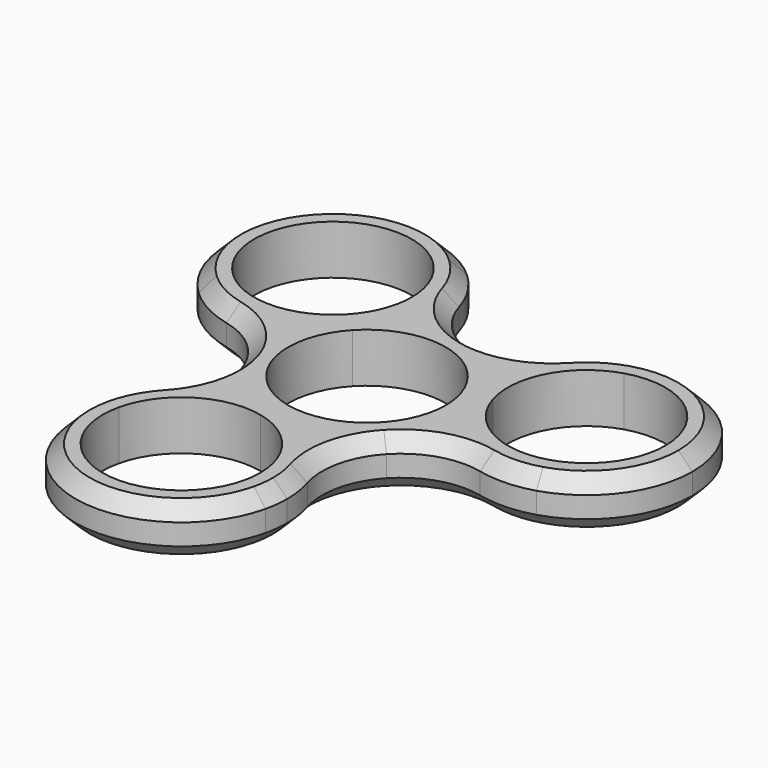
from build123d import *

# Parameters (mm, degrees)
F1_DEPTH = 7
F2_R     = 11.159
F3_SIZE  = 2


# Not quite as in the source:
# - a fillet or chamfer is up to 0.001 mm smaller than in the source, because OpenCascade refuses the exact size
# - ends of sketch curves that miss each other by under 0.0002 mm in the source are joined


with BuildPart() as f1:
    # F0 (on Top) → F1 (new body)
    with BuildSketch(Plane.XY):
        with BuildLine():
            Line((-29.35523, 6.900439), (-26.73352, 9.706189))
            ThreePointArc((-26.73352, 9.706189), (-27.268387, 25.479747), (-11.494829, 26.014613))
            Line((-11.494829, 26.014613), (-8.873119, 28.820364))
            ThreePointArc((-8.873119, 28.820364), (-30.074137, 28.101457), (-29.35523, 6.900439))
        make_face()
        with BuildLine():
            ThreePointArc((-8.873119, 28.820364), (-7.418015, 23.350137), (-4.139731, 18.735642))
            ThreePointArc((-4.139731, 18.735642), (-5.535487, 24.233724), (-8.873119, 28.820364))
        make_face()
        with BuildLine():
            ThreePointArc((-7.954175, 17.860401), (-8.732782, 13.765002), (-10.959962, 10.241056))
            ThreePointArc((-10.959962, 10.241056), (-8.01264, 12.680599), (-4.54403, 14.295167))
            ThreePointArc((-4.54403, 14.295167), (-4.222026, 16.064874), (-4.114175, 17.860401))
            ThreePointArc((-4.114175, 17.860401), (-4.120565, 18.298208), (-4.139731, 18.735642))
            ThreePointArc((-4.139731, 18.735642), (-7.418015, 23.350137), (-8.873119, 28.820364))
            Line((-8.873119, 28.820364), (-11.494829, 26.014613))
            ThreePointArc((-11.494829, 26.014613), (-8.877537, 22.305269), (-7.954175, 17.860401))
        make_face()
        with BuildLine():
            Line((-10.959962, 10.241056), (-8.154212, 7.619345))
            ThreePointArc((-8.154212, 7.619345), (-5.919925, 10.725153), (-4.54403, 14.295167))
            ThreePointArc((-4.54403, 14.295167), (-8.01264, 12.680599), (-10.959962, 10.241056))
        make_face()
        with BuildLine():
            ThreePointArc((-14.570144, 3.565235), (-11.101534, 5.179802), (-8.154212, 7.619345))
            Line((-8.154212, 7.619345), (-10.959962, 10.241056))
            ThreePointArc((-10.959962, 10.241056), (-13.19425, 7.135248), (-14.570144, 3.565235))
        make_face()
        with BuildLine():
            ThreePointArc((-14.570144, 3.565235), (-13.19425, 7.135248), (-10.959962, 10.241056))
            ThreePointArc((-10.959962, 10.241056), (-18.735967, 6.706812), (-26.73352, 9.706189))
            Line((-26.73352, 9.706189), (-29.35523, 6.900439))
            ThreePointArc((-29.35523, 6.900439), (-23.798999, 5.819232), (-18.973032, 2.861065))
            ThreePointArc((-18.973032, 2.861065), (-16.745277, 3.048638), (-14.570144, 3.565235))
        make_face()
        with BuildLine():
            ThreePointArc((-29.35523, 6.900439), (-24.553034, 3.881174), (-18.973032, 2.861065))
            ThreePointArc((-18.973032, 2.861065), (-23.798999, 5.819232), (-29.35523, 6.900439))
        make_face()
        with BuildLine():
            ThreePointArc((-20.522608, -22.094528), (-16.512804, -18.099258), (-14.155676, -12.952933))
            ThreePointArc((-14.155676, -12.952933), (-18.219277, -16.910735), (-20.522608, -22.094528))
        make_face()
        with BuildLine():
            ThreePointArc((-16.781901, -22.962121), (-11.814806, -16.013373), (-3.389033, -14.612134))
            ThreePointArc((-3.389033, -14.612134), (-6.975401, -13.27945), (-10.107962, -11.082829))
            ThreePointArc((-10.107962, -11.082829), (-12.201695, -11.86664), (-14.155676, -12.952933))
            ThreePointArc((-14.155676, -12.952933), (-16.512804, -18.099258), (-20.522608, -22.094528))
            Line((-20.522608, -22.094528), (-16.781901, -22.962121))
        make_face()
        with BuildLine():
            Line((-3.389033, -14.612134), (-2.521441, -10.871428))
            ThreePointArc((-2.521441, -10.871428), (-6.328293, -10.489382), (-10.107962, -11.082829))
            ThreePointArc((-10.107962, -11.082829), (-6.975401, -13.27945), (-3.389033, -14.612134))
        make_face()
        with BuildLine():
            ThreePointArc((4.197488, -14.400732), (1.064927, -12.204112), (-2.521441, -10.871428))
            Line((-2.521441, -10.871428), (-3.389033, -14.612134))
            ThreePointArc((-3.389033, -14.612134), (0.417819, -14.99418), (4.197488, -14.400732))
        make_face()
        with BuildLine():
            ThreePointArc((9.089526, -25.483561), (8.559988, -21.533151), (7.008761, -17.861661))
            ThreePointArc((7.008761, -17.861661), (6.859897, -23.520154), (8.70166, -28.872595))
            ThreePointArc((8.70166, -28.872595), (8.992244, -27.189139), (9.089526, -25.483561))
        make_face()
        with BuildLine():
            ThreePointArc((4.197488, -14.400732), (0.417819, -14.99418), (-3.389033, -14.612134))
            ThreePointArc((-3.389033, -14.612134), (2.826942, -18.540712), (5.249526, -25.483561))
            ThreePointArc((5.249526, -25.483561), (5.177148, -26.752511), (4.960954, -28.005002))
            Line((4.960954, -28.005002), (8.70166, -28.872595))
            ThreePointArc((8.70166, -28.872595), (6.859897, -23.520154), (7.008761, -17.861661))
            ThreePointArc((7.008761, -17.861661), (5.732441, -16.026155), (4.197488, -14.400732))
        make_face()
        with BuildLine():
            ThreePointArc((4.960954, -28.005002), (-8.431915, -36.354989), (-16.781901, -22.962121))
            Line((-16.781901, -22.962121), (-20.522608, -22.094528))
            ThreePointArc((-20.522608, -22.094528), (-9.299507, -40.095695), (8.70166, -28.872595))
            Line((8.70166, -28.872595), (4.960954, -28.005002))
        make_face()
        with BuildLine():
            ThreePointArc((-10.107962, -11.082829), (-6.328293, -10.489382), (-2.521441, -10.871428))
            ThreePointArc((-2.521441, -10.871428), (-10.675653, -3.252082), (-8.154212, 7.619345))
            ThreePointArc((-8.154212, 7.619345), (-11.101534, 5.179802), (-14.570144, 3.565235))
            ThreePointArc((-14.570144, 3.565235), (-14.99418, -0.417819), (-14.348996, -4.371078))
            ThreePointArc((-14.348996, -4.371078), (-12.680599, -8.01264), (-10.107962, -11.082829))
        make_face()
        with BuildLine():
            ThreePointArc((10.675653, 3.252082), (11.038249, 1.643976), (11.16, 0))
            ThreePointArc((11.16, 0), (6.94285, -8.737416), (-2.521441, -10.871428))
            ThreePointArc((-2.521441, -10.871428), (1.064927, -12.204112), (4.197488, -14.400732))
            ThreePointArc((4.197488, -14.400732), (7.858931, -12.776431), (10.959962, -10.241056))
            ThreePointArc((10.959962, -10.241056), (13.279449, -6.975401), (14.651993, -3.212338))
            ThreePointArc((14.651993, -3.212338), (12.248217, -0.235772), (10.675653, 3.252082))
        make_face()
        with BuildLine():
            Line((14.348996, 4.371078), (10.675653, 3.252082))
            ThreePointArc((10.675653, 3.252082), (12.248217, -0.235772), (14.651993, -3.212338))
            ThreePointArc((14.651993, -3.212338), (14.912744, -1.615567), (15, 0))
            ThreePointArc((15, 0), (14.836356, 2.209645), (14.348996, 4.371078))
        make_face()
        with BuildLine():
            ThreePointArc((10.372656, 10.835498), (10.036607, 7.02431), (10.675653, 3.252082))
            Line((10.675653, 3.252082), (14.348996, 4.371078))
            ThreePointArc((14.348996, 4.371078), (12.776431, 7.858932), (10.372656, 10.835498))
        make_face()
        with BuildLine():
            ThreePointArc((-8.154212, 7.619345), (2.521441, 10.871428), (10.675653, 3.252082))
            ThreePointArc((10.675653, 3.252082), (10.036607, 7.02431), (10.372656, 10.835498))
            ThreePointArc((10.372656, 10.835498), (7.135248, 13.19425), (3.389033, 14.612134))
            ThreePointArc((3.389033, 14.612134), (-0.59885, 14.988041), (-4.54403, 14.295167))
            ThreePointArc((-4.54403, 14.295167), (-5.919925, 10.725153), (-8.154212, 7.619345))
        make_face()
        with BuildLine():
            ThreePointArc((10.372656, 10.835498), (12.776431, 7.858932), (14.348996, 4.371078))
            ThreePointArc((14.348996, 4.371078), (15.176253, 12.872417), (21.772566, 18.298813))
            Line((21.772566, 18.298813), (20.65357, 21.972156))
            ThreePointArc((20.65357, 21.972156), (16.939103, 17.700922), (11.964271, 15.000595))
            ThreePointArc((11.964271, 15.000595), (11.012837, 12.977516), (10.372656, 10.835498))
        make_face()
        with BuildLine():
            ThreePointArc((20.65357, 21.972156), (15.637712, 19.322965), (11.964271, 15.000595))
            ThreePointArc((11.964271, 15.000595), (16.939103, 17.700922), (20.65357, 21.972156))
        make_face()
        with BuildLine():
            Line((20.65357, 21.972156), (21.772566, 18.298813))
            ThreePointArc((21.772566, 18.298813), (31.667403, 16.590848), (36.184648, 7.62316))
            ThreePointArc((36.184648, 7.62316), (33.992336, 0.980406), (28.276731, -3.052493))
            Line((28.276731, -3.052493), (29.395726, -6.725836))
            ThreePointArc((29.395726, -6.725836), (37.077992, -1.305273), (40.024648, 7.62316))
            ThreePointArc((40.024648, 7.62316), (33.953081, 19.676503), (20.65357, 21.972156))
        make_face()
        with BuildLine():
            ThreePointArc((28.276731, -3.052493), (19.775391, -2.225236), (14.348996, 4.371078))
            ThreePointArc((14.348996, 4.371078), (14.836356, 2.209645), (15, 0))
            ThreePointArc((15, 0), (14.912744, -1.615567), (14.651993, -3.212338))
            ThreePointArc((14.651993, -3.212338), (16.377659, -4.633658), (18.295407, -5.782709))
            ThreePointArc((18.295407, -5.782709), (23.930819, -5.250879), (29.395726, -6.725836))
            Line((29.395726, -6.725836), (28.276731, -3.052493))
        make_face()
        with BuildLine():
            ThreePointArc((29.395726, -6.725836), (23.930819, -5.250879), (18.295407, -5.782709))
            ThreePointArc((18.295407, -5.782709), (23.754764, -7.32299), (29.395726, -6.725836))
        make_face()
    extrude(amount=F1_DEPTH)

    # F2 (radius 11.16 in the source; OpenCascade refuses exactly that, so slightly less here)
    f2_edges = [f1.edges().sort_by_distance(p)[0] for p in [
        (-14.570144, 3.565235, 3.5),
        (-10.107962, -11.082829, 3.5),
        (10.372656, 10.835498, 3.5),
        (-4.54403, 14.295167, 3.5),
        (14.651993, -3.212338, 3.5),
        (4.197488, -14.400732, 3.5),
    ]]
    fillet(f2_edges, radius=F2_R)

    # F3
    f3_edges = [f1.edges().sort_by_distance(p)[0] for p in [
        (39.373644, 11.994238, 7),
        (39.373644, 11.994238, 0),
    ]]
    chamfer(f3_edges, length=F3_SIZE)


solid = f1.part
